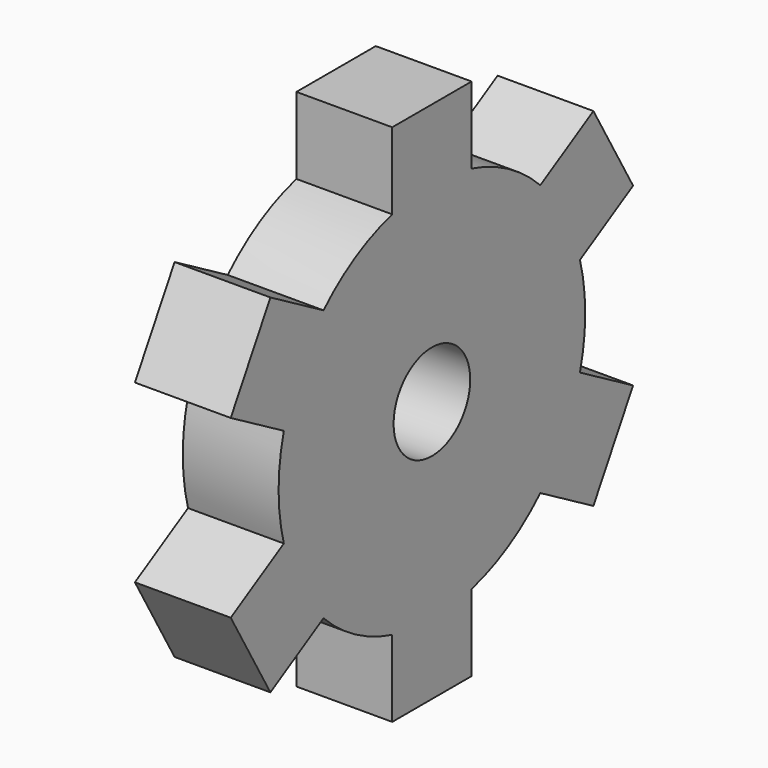
from build123d import *

# Parameters (mm, degrees)
F0_R     = 25.4
F1_DEPTH = 6.35
F3_DEPTH = 12.7
F5_COUNT = 6
F6_R     = 6.35
F7_DEPTH = 25.4


# Not quite as in the source:
# - a feature names something its author has since deleted; it is built from what else it names


with BuildPart() as f1:
    # F0 (on Right) → F1 (new body, symmetric)
    with BuildSketch(Plane.YZ):
        Circle(F0_R)
    extrude(amount=F1_DEPTH, both=True)

    # F2 (on face) → F3 (join)
    with BuildSketch(Plane.YZ.offset(6.35)):
        Polygon((6.5740037456, -24.5345159877), (0, 0), (0, -24.5345159877), align=None)
        Polygon((0, -24.5345159877), (0, 0), (-6.5740037456, -24.5345159877), align=None)
        Polygon((6.5740037456, -24.5345159877), (0, -24.5345159877), (-6.5740037456, -24.5345159877), (-6.5740037456, -34.6945159877), (6.5740037456, -34.6945159877), align=None)
    extrude(amount=-F3_DEPTH)

    # F5: F1 ×6 about axis
    f5_axis = Axis((25.0397827476, 0, 0), (1, 0, 0))


with BuildPart() as f1_1:
    add(f1.part)
    for i in range(1, F5_COUNT):
        add(f1.part.rotate(f5_axis, i * 360 / F5_COUNT))

    # F6 (on face) → F7 (cut)
    with BuildSketch(Plane(origin=(-6.35, 0, 0), x_dir=(0, -1, 0), z_dir=(-1, 0, 0))):
        Circle(F6_R)
    extrude(amount=-F7_DEPTH, mode=Mode.SUBTRACT)


solid = f1_1.part
